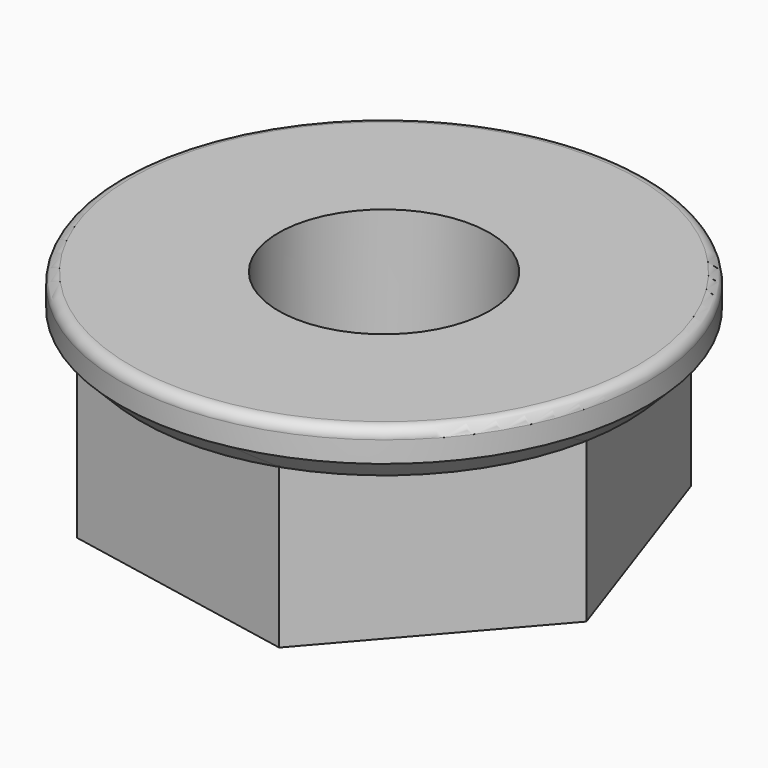
from build123d import *

# Parameters (mm, degrees)
F0_R     = 2
F1_DEPTH = 3
F2_R     = 5
F2_R_2   = 2
F3_DEPTH = 1
F5_R     = 0.2


# Not quite as in the source:
# - a fillet or chamfer that OpenCascade refuses, or shapes differently, is made with other operations: its cross-section is extruded or revolved along the edge and cut away or added


with BuildPart() as f1:
    # F0 (on Top) → F1 (new body)
    with BuildSketch(Plane.XY):
        Polygon((1.5066089403, -4.3661725612), (4.5345208255, -0.8783246648), (3.0279118852, 3.4878478965), (-1.5066089403, 4.3661725612), (-4.5345208255, 0.8783246648), (-3.0279118852, -3.4878478965), align=None)
        Circle(F0_R, mode=Mode.SUBTRACT)
    extrude(amount=F1_DEPTH)

    # F2 (on face) → F3 (join)
    with BuildSketch(Plane.XY.offset(3)):
        Circle(F2_R)
        Circle(F2_R_2, mode=Mode.SUBTRACT)
    extrude(amount=F3_DEPTH)

    # F4: chamfer of 0.4 on 1 edges, made by hand


with BuildPart() as f4_tool2:
    # F4_s3 → F4_t4 (revolve)
    with BuildSketch(Plane.XZ):
        Polygon((4.6, 3), (5, 3.4), (5, 3), align=None)
    revolve(axis=Axis((0, 0, 3), (0, 0, 1)))

    split(bisect_by=Plane(origin=(3.7812163553, 1.3047616158, 0), x_dir=(0, 0, 1), z_dir=(0.9453040888, 0.326190404, 0)), keep=Keep.TOP)


with BuildPart() as f1_1:
    add(f1.part)

    # F4_t1: cut F4_tool2
    add(f4_tool2.part, mode=Mode.SUBTRACT)


with BuildPart() as f4_tool7:
    # F4_s8 → F4_t9 (revolve)
    with BuildSketch(Plane.XZ):
        Polygon((4.6, 3), (5, 3.4), (5, 3), align=None)
    revolve(axis=Axis((0, 0, 3), (0, 0, 1)))

    split(bisect_by=Plane(origin=(0.7606514725, 3.9270102288, 0), x_dir=(0, 0, 1), z_dir=(0.1901628681, 0.9817525572, 0)), keep=Keep.TOP)


with BuildPart() as f1_2:
    add(f1_1.part)

    # F4_t6: cut F4_tool7
    add(f4_tool7.part, mode=Mode.SUBTRACT)


with BuildPart() as f4_tool12:
    # F4_s13 → F4_t14 (revolve)
    with BuildSketch(Plane.XZ):
        Polygon((4.6, 3), (5, 3.4), (5, 3), align=None)
    revolve(axis=Axis((0, 0, 3), (0, 0, 1)))

    split(bisect_by=Plane(origin=(3.0205648829, -2.622248613, 0), x_dir=(0, 0, 1), z_dir=(0.7551412207, -0.6555621532, 0)), keep=Keep.TOP)


with BuildPart() as f1_3:
    add(f1_2.part)

    # F4_t11: cut F4_tool12
    add(f4_tool12.part, mode=Mode.SUBTRACT)


with BuildPart() as f4_tool17:
    # F4_s18 → F4_t19 (revolve)
    with BuildSketch(Plane.XZ):
        Polygon((4.6, 3), (5, 3.4), (5, 3), align=None)
    revolve(axis=Axis((0, 0, 3), (0, 0, 1)))

    split(bisect_by=Plane(origin=(-3.0205648829, 2.622248613, 0), x_dir=(0, 0, 1), z_dir=(-0.7551412207, 0.6555621532, 0)), keep=Keep.TOP)


with BuildPart() as f1_4:
    add(f1_3.part)

    # F4_t16: cut F4_tool17
    add(f4_tool17.part, mode=Mode.SUBTRACT)


with BuildPart() as f4_tool22:
    # F4_s23 → F4_t24 (revolve)
    with BuildSketch(Plane.XZ):
        Polygon((4.6, 3), (5, 3.4), (5, 3), align=None)
    revolve(axis=Axis((0, 0, 3), (0, 0, 1)))

    split(bisect_by=Plane(origin=(-0.7606514725, -3.9270102288, 0), x_dir=(0, 0, 1), z_dir=(-0.1901628681, -0.9817525572, 0)), keep=Keep.TOP)


with BuildPart() as f1_5:
    add(f1_4.part)

    # F4_t21: cut F4_tool22
    add(f4_tool22.part, mode=Mode.SUBTRACT)


with BuildPart() as f4_tool27:
    # F4_s28 → F4_t29 (revolve)
    with BuildSketch(Plane.XZ):
        Polygon((4.6, 3), (5, 3.4), (5, 3), align=None)
    revolve(axis=Axis((0, 0, 3), (0, 0, 1)))

    split(bisect_by=Plane(origin=(-3.7812163553, -1.3047616158, 0), x_dir=(0, 0, 1), z_dir=(-0.9453040888, -0.326190404, 0)), keep=Keep.TOP)


with BuildPart() as f1_6:
    add(f1_5.part)

    # F4_t26: cut F4_tool27
    add(f4_tool27.part, mode=Mode.SUBTRACT)

    # F5
    f5_edges = [f1_6.edges().sort_by_distance(p)[0] for p in [
        (-5, 0, 4),
    ]]
    fillet(f5_edges, radius=F5_R)


solid = f1_6.part
